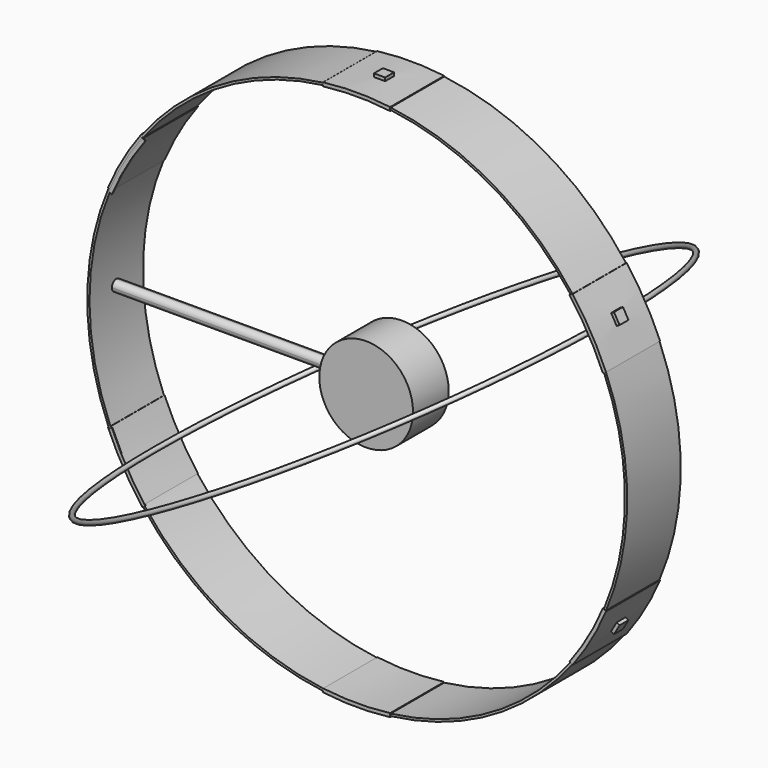
from build123d import *

# Parameters (mm, degrees)
F0_R         = 307.34
F0_R_2       = 304.8
F1_DEPTH     = 38.1
F3_DEPTH     = 76.2
F5_DEPTH     = 0.762
F7_DEPTH     = 6.35
F8_R         = 2.54
F11_DEPTH    = 6.35
F12_T1_DEPTH = 336.4838469878
F12_T3_DEPTH = 336.4838469878
F12_T5_DEPTH = 336.4838469894
F12_T7_DEPTH = 336.4838469894
F13_R        = 6.35
F14_DEPTH    = 53.34
F15_R        = 53.34
F16_DEPTH    = 25.4


# Not quite as in the source:
# - a fillet or chamfer that OpenCascade refuses, or shapes differently, is made with other operations: its cross-section is extruded or revolved along the edge and cut away or added


with BuildPart() as f1:
    # F0 (on Front) → F1 (new body, symmetric)
    with BuildSketch(Plane.XZ):
        Circle(F0_R)
        Circle(F0_R_2, mode=Mode.SUBTRACT)
    extrude(amount=F1_DEPTH, both=True)

    # F2 (on face) → F3 (join, through all)
    with BuildSketch(Plane.XZ.offset(38.1)):
        with BuildLine():
            ThreePointArc((-38.1, 304.9692863224), (0, 307.34), (38.1, 304.9692863224))
            Line((38.1, 304.9692863224), (38.1, 305.737194996))
            ThreePointArc((38.1, 305.737194996), (0, 308.102), (-38.1, 305.737194996))
            Line((-38.1, 305.737194996), (-38.1, 304.9692863224))
        make_face()
        with BuildLine():
            Line((38.1, 301.6413357682), (38.1, 302.4093748547))
            ThreePointArc((38.1, 302.4093748547), (0, 304.8), (-38.1, 302.4093748547))
            Line((-38.1, 302.4093748547), (-38.1, 301.6413357682))
            ThreePointArc((-38.1, 301.6413357682), (0, 304.038), (38.1, 301.6413357682))
        make_face()
        with BuildLine():
            Line((280.2790596067, 117.8250999999), (280.9442009667, 118.2091195432))
            ThreePointArc((280.9442009667, 118.2091195432), (263.9645430735, 152.4), (242.8442009667, 184.2002553115))
            Line((242.8442009667, 184.2002553115), (242.1790596067, 183.8162357683))
            ThreePointArc((242.1790596067, 183.8162357683), (263.3046317158, 152.019), (280.2790596067, 117.8250999999))
        make_face()
        with BuildLine():
            Line((283.1611493292, 119.489075277), (283.8261777483, 119.8730296138))
            ThreePointArc((283.8261777483, 119.8730296138), (266.8241589568, 154.051), (245.7261777483, 185.8641653822))
            Line((245.7261777483, 185.8641653822), (245.0611493292, 185.4802110454))
            ThreePointArc((245.0611493292, 185.4802110454), (266.1642475991, 153.67), (283.1611493292, 119.489075277))
        make_face()
        with BuildLine():
            Line((242.1790596067, -183.8162357683), (242.8442009667, -184.2002553115))
            ThreePointArc((242.8442009667, -184.2002553115), (263.9645430735, -152.4), (280.9442009667, -118.2091195432))
            Line((280.9442009667, -118.2091195432), (280.2790596067, -117.8250999999))
            ThreePointArc((280.2790596067, -117.8250999999), (263.3046317158, -152.019), (242.1790596067, -183.8162357683))
        make_face()
        with BuildLine():
            Line((245.0611493292, -185.4802110454), (245.7261777483, -185.8641653822))
            ThreePointArc((245.7261777483, -185.8641653822), (266.8241589568, -154.051), (283.8261777483, -119.8730296138))
            Line((283.8261777483, -119.8730296138), (283.1611493292, -119.489075277))
            ThreePointArc((283.1611493292, -119.489075277), (266.1642475991, -153.67), (245.0611493292, -185.4802110454))
        make_face()
        with BuildLine():
            Line((-38.1, -301.6413357682), (-38.1, -302.4093748547))
            ThreePointArc((-38.1, -302.4093748547), (0, -304.8), (38.1, -302.4093748547))
            Line((38.1, -302.4093748547), (38.1, -301.6413357682))
            ThreePointArc((38.1, -301.6413357682), (0, -304.038), (-38.1, -301.6413357682))
        make_face()
        with BuildLine():
            Line((-38.1, -304.9692863224), (-38.1, -305.737194996))
            ThreePointArc((-38.1, -305.737194996), (0, -308.102), (38.1, -305.737194996))
            Line((38.1, -305.737194996), (38.1, -304.9692863224))
            ThreePointArc((38.1, -304.9692863224), (0, -307.34), (-38.1, -304.9692863224))
        make_face()
        with BuildLine():
            Line((-280.2790596067, -117.8250999999), (-280.9442009667, -118.2091195432))
            ThreePointArc((-280.9442009667, -118.2091195432), (-263.9645430735, -152.4), (-242.8442009667, -184.2002553115))
            Line((-242.8442009667, -184.2002553115), (-242.1790596067, -183.8162357683))
            ThreePointArc((-242.1790596067, -183.8162357683), (-263.3046317158, -152.019), (-280.2790596067, -117.8250999999))
        make_face()
        with BuildLine():
            Line((-283.1611493292, -119.489075277), (-283.8261777483, -119.8730296138))
            ThreePointArc((-283.8261777483, -119.8730296138), (-266.8241589568, -154.051), (-245.7261777483, -185.8641653822))
            Line((-245.7261777483, -185.8641653822), (-245.0611493292, -185.4802110454))
            ThreePointArc((-245.0611493292, -185.4802110454), (-266.1642475991, -153.67), (-283.1611493292, -119.489075277))
        make_face()
        with BuildLine():
            Line((-242.1790596067, 183.8162357683), (-242.8442009667, 184.2002553115))
            ThreePointArc((-242.8442009667, 184.2002553115), (-263.9645430735, 152.4), (-280.9442009667, 118.2091195432))
            Line((-280.9442009667, 118.2091195432), (-280.2790596067, 117.8250999999))
            ThreePointArc((-280.2790596067, 117.8250999999), (-263.3046317158, 152.019), (-242.1790596067, 183.8162357683))
        make_face()
        with BuildLine():
            Line((-245.0611493292, 185.4802110454), (-245.7261777483, 185.8641653822))
            ThreePointArc((-245.7261777483, 185.8641653822), (-266.8241589568, 154.051), (-283.8261777483, 119.8730296138))
            Line((-283.8261777483, 119.8730296138), (-283.1611493292, 119.489075277))
            ThreePointArc((-283.1611493292, 119.489075277), (-266.1642475991, 153.67), (-245.0611493292, 185.4802110454))
        make_face()
    extrude(amount=-F3_DEPTH)

    # F4 (on face) → F5 (join)
    with BuildSketch(Plane.XZ.offset(38.1)):
        with BuildLine():
            Line((38.1, 301.6413357682), (38.1, 305.737194996))
            ThreePointArc((38.1, 305.737194996), (0, 308.102), (-38.1, 305.737194996))
            Line((-38.1, 305.737194996), (-38.1, 301.6413357682))
            ThreePointArc((-38.1, 301.6413357682), (0, 304.038), (38.1, 301.6413357682))
        make_face()
        with BuildLine():
            ThreePointArc((242.1790596067, 183.8162357683), (263.3046317158, 152.019), (280.2790596067, 117.8250999999))
            Line((280.2790596067, 117.8250999999), (283.8261777483, 119.8730296138))
            ThreePointArc((283.8261777483, 119.8730296138), (266.8241589568, 154.051), (245.7261777483, 185.8641653822))
            Line((245.7261777483, 185.8641653822), (242.1790596067, 183.8162357683))
        make_face()
        with BuildLine():
            ThreePointArc((280.2790596067, -117.8250999999), (263.3046317158, -152.019), (242.1790596067, -183.8162357683))
            Line((242.1790596067, -183.8162357683), (245.7261777483, -185.8641653822))
            ThreePointArc((245.7261777483, -185.8641653822), (266.8241589568, -154.051), (283.8261777483, -119.8730296138))
            Line((283.8261777483, -119.8730296138), (280.2790596067, -117.8250999999))
        make_face()
        with BuildLine():
            ThreePointArc((38.1, -301.6413357682), (0, -304.038), (-38.1, -301.6413357682))
            Line((-38.1, -301.6413357682), (-38.1, -305.737194996))
            ThreePointArc((-38.1, -305.737194996), (0, -308.102), (38.1, -305.737194996))
            Line((38.1, -305.737194996), (38.1, -301.6413357682))
        make_face()
        with BuildLine():
            ThreePointArc((-240.6272865628, -184.7121523529), (-261.7528586719, -152.9149165846), (-278.7272865628, -118.7210165845))
            Line((-278.7272865628, -118.7210165845), (-282.2744047044, -120.7689461984))
            ThreePointArc((-282.2744047044, -120.7689461984), (-265.2723859129, -154.9469165846), (-244.1744047044, -186.7600819668))
            Line((-244.1744047044, -186.7600819668), (-240.6272865628, -184.7121523529))
        make_face()
        with BuildLine():
            ThreePointArc((-278.7272865628, 115.1373502461), (-261.7528586719, 149.3312502462), (-240.6272865628, 181.1284860145))
            Line((-240.6272865628, 181.1284860145), (-244.1744047044, 183.1764156284))
            ThreePointArc((-244.1744047044, 183.1764156284), (-265.2723859129, 151.3632502462), (-282.2744047044, 117.18527986))
            Line((-282.2744047044, 117.18527986), (-278.7272865628, 115.1373502461))
        make_face()
    extrude(amount=F5_DEPTH)

    # F6 (on Front) → F7 (join, symmetric)
    with BuildSketch(Plane.XZ):
        with BuildLine():
            ThreePointArc((-6.35, 308.0365561163), (0, 308.102), (6.35, 308.0365561163))
            Line((6.35, 308.0365561163), (6.35, 311.8465561163))
            Line((6.35, 311.8465561163), (-6.35, 311.8465561163))
            Line((-6.35, 311.8465561163), (-6.35, 308.0365561163))
        make_face()
        with BuildLine():
            ThreePointArc((263.592482891, 159.5175393722), (266.8241589568, 154.051), (269.942482891, 148.5190167441))
            Line((269.942482891, 148.5190167441), (273.2420396794, 150.4240167441))
            Line((273.2420396794, 150.4240167441), (266.8920396794, 161.4225393722))
            Line((266.8920396794, 161.4225393722), (263.592482891, 159.5175393722))
        make_face()
        with BuildLine():
            ThreePointArc((269.942482891, -148.5190167441), (266.8241589568, -154.051), (263.592482891, -159.5175393722))
            Line((263.592482891, -159.5175393722), (266.8920396794, -161.4225393722))
            Line((266.8920396794, -161.4225393722), (273.2420396794, -150.4240167441))
            Line((273.2420396794, -150.4240167441), (269.942482891, -148.5190167441))
        make_face()
        with BuildLine():
            ThreePointArc((6.35, -308.0365561163), (0, -308.102), (-6.35, -308.0365561163))
            Line((-6.35, -308.0365561163), (-6.35, -311.8465561163))
            Line((-6.35, -311.8465561163), (6.35, -311.8465561163))
            Line((6.35, -311.8465561163), (6.35, -308.0365561163))
        make_face()
        with BuildLine():
            ThreePointArc((-263.592482891, -159.5175393722), (-266.8241589568, -154.051), (-269.942482891, -148.5190167441))
            Line((-269.942482891, -148.5190167441), (-273.2420396794, -150.4240167441))
            Line((-273.2420396794, -150.4240167441), (-266.8920396794, -161.4225393722))
            Line((-266.8920396794, -161.4225393722), (-263.592482891, -159.5175393722))
        make_face()
        with BuildLine():
            ThreePointArc((-269.942482891, 148.5190167441), (-266.8241589568, 154.051), (-263.592482891, 159.5175393722))
            Line((-263.592482891, 159.5175393722), (-266.8920396794, 161.4225393722))
            Line((-266.8920396794, 161.4225393722), (-273.2420396794, 150.4240167441))
            Line((-273.2420396794, 150.4240167441), (-269.942482891, 148.5190167441))
        make_face()
    extrude(amount=F7_DEPTH, both=True)


with BuildPart() as f9:
    # F8 (on Front) → F9 (revolve)
    with BuildSketch(Plane.XZ):
        with Locations((261.1049271902, 150.749)):
            Circle(F8_R)
    revolve(axis=Axis((-61.2589323324, 0, 106.1035832171), (-0.5, 0, 0.8660254038)))


with BuildPart() as f11:
    # F10 (on Front) → F11 (new body, symmetric)
    with BuildSketch(Plane.XZ):
        with BuildLine():
            Line((0, 6.3499999233), (-304.7338469894, 6.3499999233))
            ThreePointArc((-304.7338469894, 6.3499999233), (-304.8, -3.84e-08), (-304.7338469878, -6.35))
            Line((-304.7338469878, -6.35), (0, -6.35))
            Line((0, -6.35), (0, 6.3499999233))
        make_face()
    extrude(amount=F11_DEPTH, both=True)

    # F12: fillet of radius 6.35 on 4 edges, made by hand

    # F12_s2 → F12_t1 (cut)
    with BuildSketch(Plane.YZ.offset(-320.6088469878)):
        with BuildLine():
            ThreePointArc((0, -6.35), (4.4901280605, -4.4901280605), (6.35, 0))
            Line((6.35, 0), (6.35, -6.35))
            Line((6.35, -6.35), (0, -6.35))
        make_face()
    extrude(amount=F12_T1_DEPTH, mode=Mode.SUBTRACT)

    # F12_s4 → F12_t3 (cut)
    with BuildSketch(Plane.YZ.offset(-320.6088469878)):
        with BuildLine():
            ThreePointArc((0, -6.35), (-4.4901280605, -4.4901280605), (-6.35, 0))
            Line((-6.35, 0), (-6.35, -6.35))
            Line((-6.35, -6.35), (0, -6.35))
        make_face()
    extrude(amount=F12_T3_DEPTH, mode=Mode.SUBTRACT)

    # F12_s6 → F12_t5 (cut)
    with BuildSketch(Plane.YZ.offset(-320.6088469894)):
        with BuildLine():
            ThreePointArc((6.35, -7.67e-08), (4.4901280605, 4.4901279838), (0, 6.3499999233))
            Line((0, 6.3499999233), (6.35, 6.3499999233))
            Line((6.35, 6.3499999233), (6.35, -7.67e-08))
        make_face()
    extrude(amount=F12_T5_DEPTH, mode=Mode.SUBTRACT)

    # F12_s8 → F12_t7 (cut)
    with BuildSketch(Plane.YZ.offset(-320.6088469894)):
        with BuildLine():
            ThreePointArc((0, 6.3499999233), (-4.4901280605, 4.4901279838), (-6.35, -7.67e-08))
            Line((-6.35, -7.67e-08), (-6.35, 6.3499999233))
            Line((-6.35, 6.3499999233), (0, 6.3499999233))
        make_face()
    extrude(amount=F12_T7_DEPTH, mode=Mode.SUBTRACT)

    # F13 (on face) → F14 (cut)
    with BuildSketch(Plane.YZ):
        with Locations((0, -7.67e-08)):
            Circle(F13_R)
    extrude(amount=-F14_DEPTH, mode=Mode.SUBTRACT)


with BuildPart() as f16:
    # F15 (on Front) → F16 (new body, symmetric)
    with BuildSketch(Plane.XZ):
        Circle(F15_R)
    extrude(amount=F16_DEPTH, both=True)


solid = Compound([f1.part, f9.part, f11.part, f16.part])
